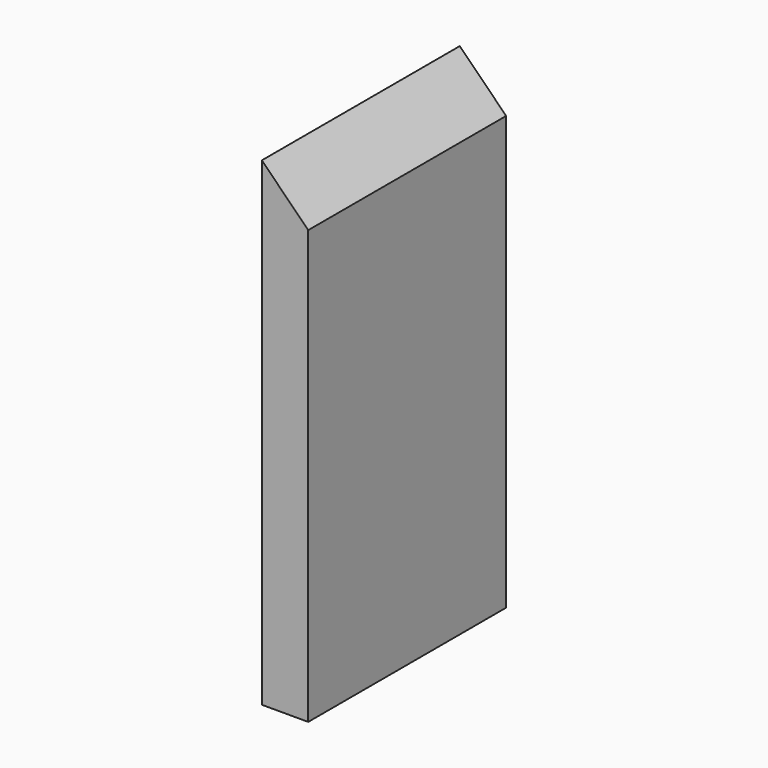
from build123d import *

# Parameters (mm, degrees)
F0_W     = 101.6
F0_H     = 196.85
F1_DEPTH = 19.05
F2_SIZE  = 19.04999


# Not quite as in the source:
# - a fillet or chamfer is up to 0.001 mm smaller than in the source, because OpenCascade refuses the exact size


with BuildPart() as f1:
    # F0 (on Right) → F1 (new body)
    with BuildSketch(Plane.YZ):
        with Locations((-6.1650511805, 0)):
            Rectangle(F0_W, F0_H)
    extrude(amount=F1_DEPTH)

    # F2 (size 19.05 in the source; OpenCascade refuses exactly that, so slightly less here)
    f2_edges = [f1.edges().sort_by_distance(p)[0] for p in [
        (19.05, -6.165051, 98.425),
    ]]
    chamfer(f2_edges, length=F2_SIZE)


solid = f1.part
